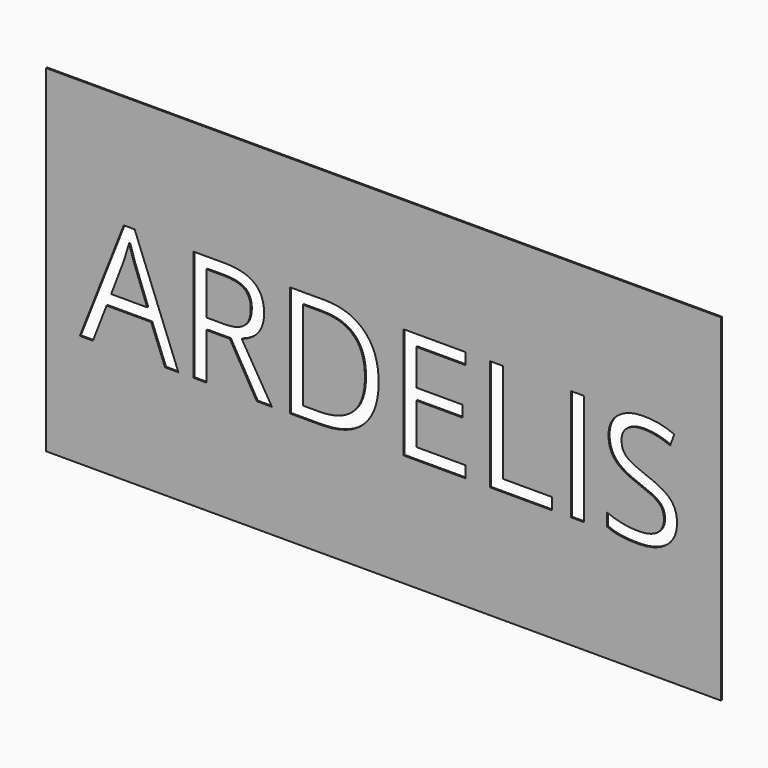
from build123d import *

# Parameters (mm, degrees)
F0_W         = 1000
F0_H         = 500
F1_DEPTH     = 2
F2_TEXT_SIZE = 230.7877233753
F3_DEPTH     = 2


# Not quite as in the source:
# - Text() gives the source's letters only with a copy of the font that has no kerning and outlines rounded to 1/6400 em; it was checked with that copy


with BuildPart() as f1:
    # F0 (on Front) → F1 (new body)
    with BuildSketch(Plane.XZ):
        Rectangle(F0_W, F0_H)
    extrude(amount=F1_DEPTH)

    # F2 (on face) → F3 (cut)
    with BuildSketch(Plane.XZ.offset(2)):
        with Locations((-450, -83.1671608302)):
            Text('ARDELIS', F2_TEXT_SIZE, font='Open Sans', text_align=(TextAlign.LEFT, TextAlign.BOTTOM))
    extrude(amount=-F3_DEPTH, mode=Mode.SUBTRACT)


solid = f1.part
